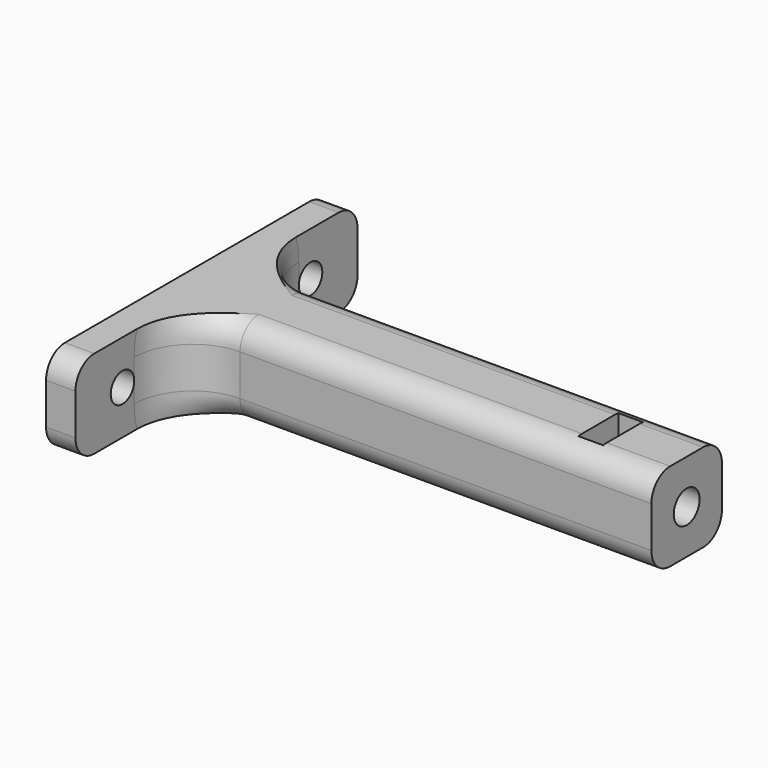
from build123d import *

# Parameters (mm, degrees)
F1_DEPTH     = 15
F3_D         = 5.5
F3_DEPTH     = 21
F3_TIP       = 1.6523667023
F5_D         = 5
F6_R         = 4
F7_T1_DEPTH  = 7
F7_T6_ANGLE  = 359.64
F7_T12_ANGLE = 359.64
F7_T18_ANGLE = 359.64
F7_T24_ANGLE = 359.64
F10_DEPTH    = 4.2


# Not quite as in the source:
# - a fillet or chamfer that OpenCascade refuses, or shapes differently, is made with other operations: its cross-section is extruded or revolved along the edge and cut away or added


with BuildPart() as f1:
    # F0 (on Top) → F1 (new body)
    with BuildSketch(Plane.XY):
        Polygon((-17.3867209846, 30), (-22.3867209846, 30), (-22.3867209846, -30), (-17.3867209846, -30), (-17.3867209846, -7.5), (62.6132790154, -7.5), (62.6132790154, 7.5), (-17.3867209846, 7.5), align=None)
    extrude(amount=F1_DEPTH)

    # F3
    with Locations(Plane.YZ.offset(62.6132790154)):
        with Locations((0, 7.5)):
            Hole(F3_D / 2, depth=F3_DEPTH)
            with Locations((0, 0, -(F3_DEPTH + F3_TIP / 2))):  # 118° drill point
                Cone(0, F3_D / 2, F3_TIP, mode=Mode.SUBTRACT)

    # F5 (through all)
    with Locations(Plane.YZ.offset(-17.3867209846)):
        with Locations((-20, 7.5), (20, 7.5)):
            Hole(F5_D / 2)

    # F6
    f6_edges = [f1.edges().sort_by_distance(p)[0] for p in [
        (22.613279, -7.5, 15),
        (22.613279, 7.5, 15),
        (22.613279, -7.5, 0),
        (22.613279, 7.5, 0),
        (-19.886721, -30, 15),
        (-19.886721, -30, 0),
        (-19.886721, 30, 15),
        (-19.886721, 30, 0),
    ]]
    fillet(f6_edges, radius=F6_R)

    # F7: fillet of radius 10 on 2 edges, made by hand

    # F7_s2 → F7_t1 (join)
    with BuildSketch(Plane.XY.offset(4)):
        with BuildLine():
            ThreePointArc((-17.3867209846, -17.5), (-14.4577887965, -10.4289321881), (-7.3867209846, -7.5))
            Line((-7.3867209846, -7.5), (-17.3867209846, -7.5))
            Line((-17.3867209846, -7.5), (-17.3867209846, -17.5))
        make_face()
        with BuildLine():
            ThreePointArc((-17.3867209846, 17.5), (-14.4577887965, 10.4289321881), (-7.3867209846, 7.5))
            Line((-7.3867209846, 7.5), (-17.3867209846, 7.5))
            Line((-17.3867209846, 7.5), (-17.3867209846, 17.5))
        make_face()
    extrude(amount=F7_T1_DEPTH)


with BuildPart() as f7_tool4:
    # F7_s5 → F7_t6 (revolve)
    with BuildSketch(Plane(origin=(0, -0.0249939071, 3.9778515186), x_dir=(1, 0, 0), z_dir=(0, 0.006283144, -0.9999802609))):
        with BuildLine():
            ThreePointArc((-17.3867209846, -17.5250634889), (-14.4577887965, -10.453995677), (-7.3867209846, -7.5250634889))
            Line((-7.3867209846, -7.5250634889), (-17.3867209846, -7.5250634889))
            Line((-17.3867209846, -7.5250634889), (-17.3867209846, -17.5250634889))
        make_face()
    revolve(axis=Axis((-17.3867209846, 3.5, 4), (1, 0, 0)), revolution_arc=F7_T6_ANGLE)

    split(bisect_by=Plane.XY, keep=Keep.TOP)

    split(bisect_by=Plane.XY.offset(15), keep=Keep.BOTTOM)


with BuildPart() as f1_1:
    add(f1.part)

    # F7_t3: union F7_tool4
    add(f7_tool4.part)


with BuildPart() as f7_tool10:
    # F7_s11 → F7_t12 (revolve)
    with BuildSketch(Plane(origin=(0, 0.069251392, 11.0215563129), x_dir=(1, 0, 0), z_dir=(0, 0.006283144, 0.9999802609))):
        with BuildLine():
            ThreePointArc((-17.3867209846, 17.4308163294), (-14.4577887965, 10.3597485175), (-7.3867209846, 7.4308163294))
            Line((-7.3867209846, 7.4308163294), (-17.3867209846, 7.4308163294))
            Line((-17.3867209846, 7.4308163294), (-17.3867209846, 17.4308163294))
        make_face()
    revolve(axis=Axis((-17.3867209846, 3.5, 11), (-1, 0, 0)), revolution_arc=F7_T12_ANGLE)

    split(bisect_by=Plane.XY, keep=Keep.TOP)

    split(bisect_by=Plane.XY.offset(15), keep=Keep.BOTTOM)


with BuildPart() as f1_2:
    add(f1_1.part)

    # F7_t9: union F7_tool10
    add(f7_tool10.part)


with BuildPart() as f7_tool16:
    # F7_s17 → F7_t18 (revolve)
    with BuildSketch(Plane(origin=(0, 0.0249939071, 3.9778515186), x_dir=(1, 0, 0), z_dir=(0, -0.006283144, -0.9999802609))):
        with BuildLine():
            ThreePointArc((-17.3867209846, 17.5250634889), (-14.4577887965, 10.453995677), (-7.3867209846, 7.5250634889))
            Line((-7.3867209846, 7.5250634889), (-17.3867209846, 7.5250634889))
            Line((-17.3867209846, 7.5250634889), (-17.3867209846, 17.5250634889))
        make_face()
    revolve(axis=Axis((-17.3867209846, -3.5, 4), (-1, 0, 0)), revolution_arc=F7_T18_ANGLE)

    split(bisect_by=Plane.XY, keep=Keep.TOP)

    split(bisect_by=Plane.XY.offset(15), keep=Keep.BOTTOM)


with BuildPart() as f1_3:
    add(f1_2.part)

    # F7_t15: union F7_tool16
    add(f7_tool16.part)


with BuildPart() as f7_tool22:
    # F7_s23 → F7_t24 (revolve)
    with BuildSketch(Plane(origin=(0, -0.069251392, 11.0215563129), x_dir=(1, 0, 0), z_dir=(0, -0.006283144, 0.9999802609))):
        with BuildLine():
            ThreePointArc((-17.3867209846, -17.4308163294), (-14.4577887965, -10.3597485175), (-7.3867209846, -7.4308163294))
            Line((-7.3867209846, -7.4308163294), (-17.3867209846, -7.4308163294))
            Line((-17.3867209846, -7.4308163294), (-17.3867209846, -17.4308163294))
        make_face()
    revolve(axis=Axis((-17.3867209846, -3.5, 11), (1, 0, 0)), revolution_arc=F7_T24_ANGLE)

    split(bisect_by=Plane.XY, keep=Keep.TOP)

    split(bisect_by=Plane.XY.offset(15), keep=Keep.BOTTOM)


with BuildPart() as f1_4:
    add(f1_3.part)

    # F7_t21: union F7_tool22
    add(f7_tool22.part)

    # F9 (on offset) → F10 (cut)
    with BuildSketch(Plane.YZ.offset(47.6132790154)):
        Polygon((0, 2.5925227119), (4.25, 5.0462613559), (4.25, 9.9537386441), (4.25, 17.4553611223), (-4.25, 17.4553611223), (-4.25, 9.9537386441), (-4.25, 5.0462613559), align=None)
    extrude(amount=F10_DEPTH, mode=Mode.SUBTRACT)


solid = f1_4.part
